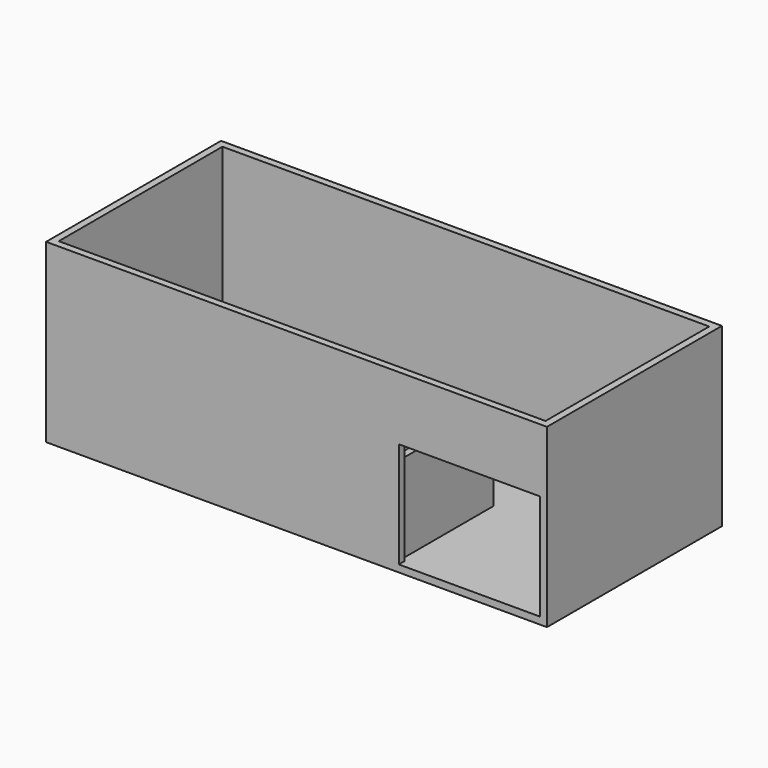
from build123d import *

# Parameters (mm, degrees)
F0_W     = 142
F0_H     = 62
F1_DEPTH = 50
F2_W     = 138
F2_H     = 58
F3_DEPTH = 48
F6_W     = 40
F6_H     = 30
F7_DEPTH = 2
F8_W     = 2
F8_H     = 33
F9_DEPTH = 25


# Not quite as in the source:
# - a feature names something its author has since deleted; it is built from what else it names


with BuildPart() as f1:
    # F0 (on Top) → F1 (new body)
    with BuildSketch(Plane.XY):
        with Locations((34.9231133461, -3.5940962459)):
            Rectangle(F0_W, F0_H)
    extrude(amount=F1_DEPTH)

    # F2 (on face) → F3 (cut)
    with BuildSketch(Plane.XY.offset(50)):
        with Locations((34.9231133461, -3.5940962459)):
            Rectangle(F2_W, F2_H)
    extrude(amount=-F3_DEPTH, mode=Mode.SUBTRACT)

    # F6 (on face) → F7 (cut)
    with BuildSketch(Plane.XZ.offset(34.5940962459)):
        with Locations((83.9231133461, 17)):
            Rectangle(F6_W, F6_H)
    extrude(amount=-F7_DEPTH, mode=Mode.SUBTRACT)

    # F8 (on face) → F9 (join)
    with BuildSketch(Plane.XY.offset(2)):
        with Locations((61.7997199297, -16.0940962459)):
            Rectangle(F8_W, F8_H)
    extrude(amount=F9_DEPTH)


solid = f1.part
